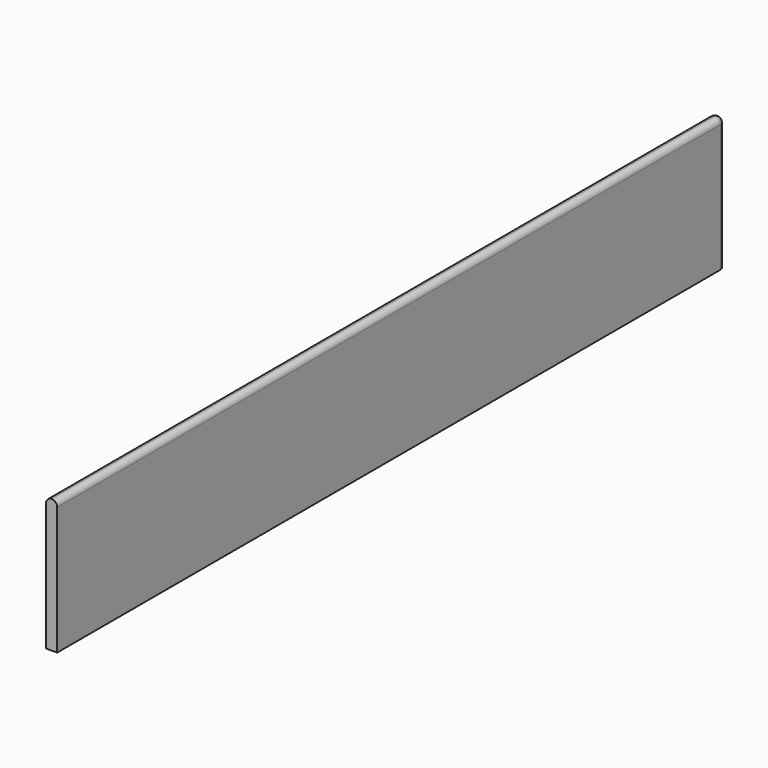
from build123d import *

# Parameters (mm, degrees)
F0_W     = 750
F0_H     = 120
F1_DEPTH = 10
F2_R     = 4.99999


# Not quite as in the source:
# - a fillet or chamfer is up to 0.001 mm smaller than in the source, because OpenCascade refuses the exact size


with BuildPart() as f1:
    # F0 (on Right) → F1 (new body)
    with BuildSketch(Plane.YZ):
        Rectangle(F0_W, F0_H)
    extrude(amount=F1_DEPTH)

    # F2 (radius 5 in the source; OpenCascade refuses exactly that, so slightly less here)
    f2_edges = [f1.edges().sort_by_distance(p)[0] for p in [
        (10, 375, 0),
        (5, 375, 60),
        (0, 375, 0),
        (0, 0, 60),
        (10, 0, 60),
    ]]
    fillet(f2_edges, radius=F2_R)


solid = f1.part
